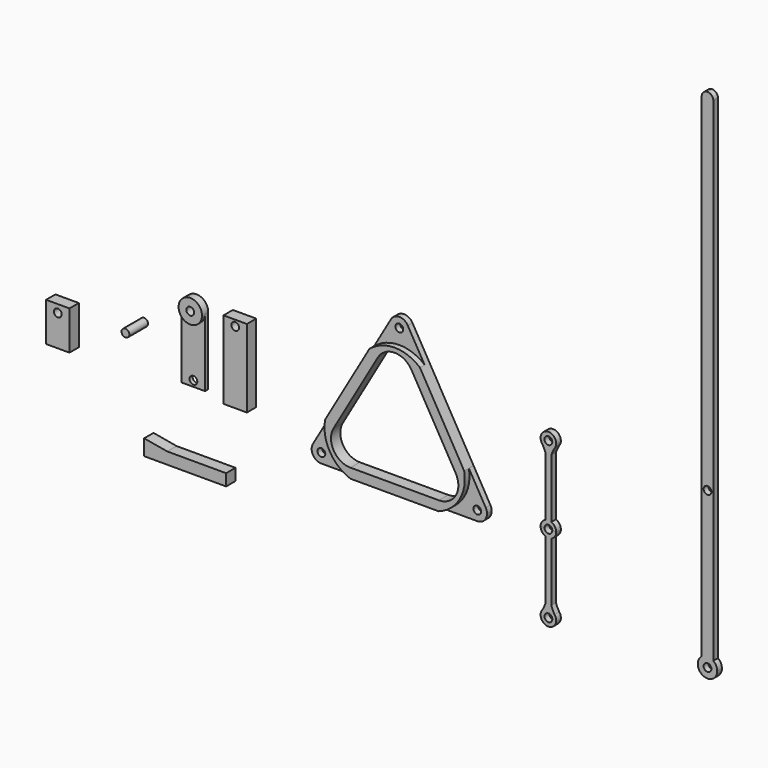
from build123d import *
from build123d import SkipClean  # not in build123d's __all__

# Parameters (mm, degrees)
F1_DEPTH  = 3
F0_R      = 1
F2_DEPTH  = 1.5
F4_DEPTH  = 1.5
F3_R      = 1
F5_DEPTH  = 1.5
F7_W      = 6
F7_H      = 20
F7_R      = 1
F8_DEPTH  = 3
F9_DEPTH  = 6
F10_DEPTH = 2
F11_DEPTH = 1
F12_R     = 1
F13_DEPTH = 1.5
F7_H_2    = 10
F14_DEPTH = 3
F16_DEPTH = 3


with BuildPart() as f1:
    # F0 (on Front) → F1 (new body)
    with BuildSketch(Plane.XZ):
        with BuildLine():
            Line((-33.1328085528, 8.75), (-44.4725545149, 28.3910161514))
            ThreePointArc((-44.4725545149, 28.3910161514), (-50.9677450433, 30.7875629885), (-57.4629355717, 28.3910161514))
            Line((-57.4629355717, 28.3910161514), (-68.8026815338, 8.75))
            ThreePointArc((-68.8026815338, 8.75), (-67.630556712, 1.9267265814), (-62.3074910055, -2.5))
            Line((-62.3074910055, -2.5), (-39.7018864751, -2.5))
            ThreePointArc((-39.7018864751, -2.5), (-34.3340694771, 1.9085363771), (-33.1328085528, 8.75))
        make_face()
        with BuildLine():
            Line((-39.6279990812, 0), (-62.3074910055, 0))
            ThreePointArc((-62.3074910055, 0), (-66.6376180244, 2.5), (-66.6376180244, 7.5))
            Line((-66.6376180244, 7.5), (-55.2978720622, 27.1410161514))
            ThreePointArc((-55.2978720622, 27.1410161514), (-50.9677450433, 29.6410161514), (-46.6376180244, 27.1410161514))
            Line((-46.6376180244, 27.1410161514), (-35.2978720622, 7.5))
            ThreePointArc((-35.2978720622, 7.5), (-35.2978720622, 2.5), (-39.6279990812, 0))
        make_face(mode=Mode.SUBTRACT)
    extrude(amount=F1_DEPTH)

    # F0 (on Front) → F2 (join)
    with BuildSketch(Plane.XZ):
        with BuildLine():
            ThreePointArc((-53.1328085528, 35.8910161514), (-51.6147926561, 32.2262015857), (-48.4677450433, 34.6410161514))
            ThreePointArc((-48.4677450433, 34.6410161514), (-48.5529304776, 35.2880637641), (-48.8026815338, 35.8910161514))
            ThreePointArc((-48.8026815338, 35.8910161514), (-50.9677450433, 37.1410161514), (-53.1328085528, 35.8910161514))
        make_face()
        with Locations((-50.9677450433, 34.6410161514)):
            Circle(F0_R, mode=Mode.SUBTRACT)
        with BuildLine():
            ThreePointArc((-48.8026815338, 35.8910161514), (-48.5529304776, 35.2880637641), (-48.4677450433, 34.6410161514))
            ThreePointArc((-48.4677450433, 34.6410161514), (-51.6147926561, 32.2262015857), (-53.1328085528, 35.8910161514))
            Line((-53.1328085528, 35.8910161514), (-57.4629355717, 28.3910161514))
            ThreePointArc((-57.4629355717, 28.3910161514), (-50.9677450433, 30.7875629885), (-44.4725545149, 28.3910161514))
            Line((-44.4725545149, 28.3910161514), (-48.8026815338, 35.8910161514))
        make_face()
        with BuildLine():
            Line((-28.8026815338, 1.25), (-33.1328085528, 8.75))
            ThreePointArc((-33.1328085528, 8.75), (-34.3340694771, 1.9085363771), (-39.7018864751, -2.5))
            Line((-39.7018864751, -2.5), (-30.9677450433, -2.5))
            ThreePointArc((-30.9677450433, -2.5), (-33.1328085528, 1.25), (-28.8026815338, 1.25))
        make_face()
        with BuildLine():
            ThreePointArc((-28.4677450433, 0), (-28.5529304776, 0.6470476128), (-28.8026815338, 1.25))
            ThreePointArc((-28.8026815338, 1.25), (-33.1328085528, 1.25), (-30.9677450433, -2.5))
            ThreePointArc((-30.9677450433, -2.5), (-29.1999780903, -1.767766953), (-28.4677450433, 0))
        make_face()
        with Locations((-30.9677450433, 0)):
            Circle(F0_R, mode=Mode.SUBTRACT)
        with BuildLine():
            ThreePointArc((-62.3074910055, -2.5), (-67.630556712, 1.9267265814), (-68.8026815338, 8.75))
            Line((-68.8026815338, 8.75), (-73.1328085528, 1.25))
            ThreePointArc((-73.1328085528, 1.25), (-70.3206974306, 2.4148145657), (-68.4677450433, 0))
            ThreePointArc((-68.4677450433, 0), (-69.1999780903, -1.767766953), (-70.9677450433, -2.5))
            Line((-70.9677450433, -2.5), (-62.3074910055, -2.5))
        make_face()
        with BuildLine():
            ThreePointArc((-68.4677450433, 0), (-70.3206974306, 2.4148145657), (-73.1328085528, 1.25))
            ThreePointArc((-73.1328085528, 1.25), (-73.1328085528, -1.25), (-70.9677450433, -2.5))
            ThreePointArc((-70.9677450433, -2.5), (-69.1999780903, -1.767766953), (-68.4677450433, 0))
        make_face()
        with Locations((-70.9677450433, 0)):
            Circle(F0_R, mode=Mode.SUBTRACT)
    extrude(amount=F2_DEPTH)


with BuildPart() as f4:
    # F3 (on Front) → F4 (new body)
    with BuildSketch(Plane.XZ):
        with BuildLine():
            Line((-11.9925050726, 18.5729119312), (-13.4582213502, 18.5729119312))
            Line((-13.4582213502, 18.5729119312), (-13.4582213502, 3.4791482928))
            ThreePointArc((-13.4582213502, 3.4791482928), (-14.3784990615, 2.7439302749), (-14.7253632114, 1.6182563162))
            Line((-14.7253632114, 1.6182563162), (-13.7253632114, 1.6182563162))
            ThreePointArc((-13.7253632114, 1.6182563162), (-12.7253632114, 2.6182563162), (-11.7253632114, 1.6182563162))
            Line((-11.7253632114, 1.6182563162), (-10.7253632114, 1.6182563162))
            ThreePointArc((-10.7253632114, 1.6182563162), (-11.0722273613, 2.7439302749), (-11.9925050726, 3.4791482928))
            Line((-11.9925050726, 3.4791482928), (-11.9925050726, 18.5729119312))
        make_face()
    extrude(amount=F4_DEPTH)

    # F3 (on Front) → F5 (join)
    with BuildSketch(Plane.XZ):
        with BuildLine():
            ThreePointArc((-14.3201244522, 20.4113028852), (-13.8423935019, 19.5140392553), (-13.4582213502, 18.5729119312))
            Line((-13.4582213502, 18.5729119312), (-11.9925050726, 18.5729119312))
            ThreePointArc((-11.9925050726, 18.5729119312), (-11.6083329209, 19.5140392553), (-11.1306019706, 20.4113028852))
            ThreePointArc((-11.1306019706, 20.4113028852), (-12.7253632114, 23.6182563162), (-14.3201244522, 20.4113028852))
        make_face()
        with Locations((-12.7253632114, 21.6182563162)):
            Circle(F3_R, mode=Mode.SUBTRACT)
    extrude(amount=F5_DEPTH)

    # F6: F4 across face


with BuildPart() as f4_1:
    add(f4.part, clean=False)
    with SkipClean():  # cleaning this boolean's faces spoils the solid; the shape is the same uncleaned
        add(f4.part.mirror(Plane(origin=(-14.2253632114, -0.75, 1.6182563162), x_dir=(1, 0, 0), z_dir=(0, 0, -1))), clean=False)


with BuildPart() as f8:
    # F7 (on Front) → F8 (new body)
    with BuildSketch(Plane.XZ):
        with Locations((-91.8792099953, 13.8065970875)):
            Rectangle(F7_W, F7_H)
        with Locations((-91.8792099953, 22.3065970875)):
            Circle(F7_R, mode=Mode.SUBTRACT)
    extrude(amount=F8_DEPTH)


with BuildPart() as f9:
    # F7 (on Front) → F9 (new body)
    with BuildSketch(Plane.XZ):
        with Locations((-117.6395714283, 13.6291719973)):
            Circle(F7_R)
    extrude(amount=F9_DEPTH)


with BuildPart() as f10:
    # F7 (on Front) → F10 (new body)
    with BuildSketch(Plane.XZ):
        with BuildLine():
            ThreePointArc((-107.204214007, 21.3065970875), (-104.204214007, 18.3065970875), (-101.204214007, 21.3065970875))
            Line((-101.204214007, 21.3065970875), (-103.204214007, 21.3065970875))
            ThreePointArc((-103.204214007, 21.3065970875), (-104.204214007, 20.3065970875), (-105.204214007, 21.3065970875))
            Line((-105.204214007, 21.3065970875), (-107.204214007, 21.3065970875))
        make_face()
        with BuildLine():
            Line((-103.204214007, 21.3065970875), (-101.204214007, 21.3065970875))
            ThreePointArc((-101.204214007, 21.3065970875), (-104.204214007, 24.3065970875), (-107.204214007, 21.3065970875))
            Line((-107.204214007, 21.3065970875), (-105.204214007, 21.3065970875))
            ThreePointArc((-105.204214007, 21.3065970875), (-104.204214007, 22.3065970875), (-103.204214007, 21.3065970875))
        make_face()
    extrude(amount=F10_DEPTH)

    # F7 (on Front) → F11 (join)
    with BuildSketch(Plane.XZ):
        with BuildLine():
            Line((-101.204214007, 3.8065970875), (-101.204214007, 21.3065970875))
            ThreePointArc((-101.204214007, 21.3065970875), (-104.204214007, 18.3065970875), (-107.204214007, 21.3065970875))
            Line((-107.204214007, 21.3065970875), (-107.204214007, 3.8065970875))
            Line((-107.204214007, 3.8065970875), (-101.204214007, 3.8065970875))
        make_face()
        with Locations((-104.204214007, 5.3065970875)):
            Circle(F7_R, mode=Mode.SUBTRACT)
    extrude(amount=F11_DEPTH)


with BuildPart() as f13:
    # F12 (on Front) → F13 (new body)
    with BuildSketch(Plane.XZ):
        with BuildLine():
            ThreePointArc((26.5937472323, -14.345602423), (28.0937472323, -13.845602423), (29.5937472323, -14.345602423))
            Line((29.5937472323, -14.345602423), (29.5937472323, 112.154397577))
            ThreePointArc((29.5937472323, 112.154397577), (29.1544074041, 113.2150577488), (28.0937472323, 113.654397577))
            ThreePointArc((28.0937472323, 113.654397577), (27.0330870605, 113.2150577488), (26.5937472323, 112.154397577))
            Line((26.5937472323, 112.154397577), (26.5937472323, -14.345602423))
        make_face()
        with Locations((28.0937472323, 23.654397577)):
            Circle(F12_R, mode=Mode.SUBTRACT)
        with BuildLine():
            Line((29.5937472323, -14.345602423), (29.5937472323, -16.345602423))
            Line((29.5937472323, -16.345602423), (29.0937472323, -16.345602423))
            ThreePointArc((29.0937472323, -16.345602423), (28.0937472323, -17.345602423), (27.0937472323, -16.345602423))
            Line((27.0937472323, -16.345602423), (26.5937472323, -16.345602423))
            Line((26.5937472323, -16.345602423), (26.5937472323, -14.345602423))
            ThreePointArc((26.5937472323, -14.345602423), (26.9757132436, -18.5816704005), (30.5937472323, -16.345602423))
            ThreePointArc((30.5937472323, -16.345602423), (30.3298152098, -15.2275684342), (29.5937472323, -14.345602423))
        make_face()
        with BuildLine():
            Line((29.0937472323, -16.345602423), (29.5937472323, -16.345602423))
            Line((29.5937472323, -16.345602423), (29.5937472323, -14.345602423))
            ThreePointArc((29.5937472323, -14.345602423), (28.0937472323, -13.845602423), (26.5937472323, -14.345602423))
            Line((26.5937472323, -14.345602423), (26.5937472323, -16.345602423))
            Line((26.5937472323, -16.345602423), (27.0937472323, -16.345602423))
            ThreePointArc((27.0937472323, -16.345602423), (28.0937472323, -15.345602423), (29.0937472323, -16.345602423))
        make_face()
    extrude(amount=F13_DEPTH)


with BuildPart() as f14:
    # F7 (on Front) → F14 (new body)
    with BuildSketch(Plane.XZ):
        with Locations((-137.3983682394, 7.5233563501)):
            Rectangle(F7_W, F7_H_2)
        with Locations((-137.3983682394, 10.5233563501)):
            Circle(F7_R, mode=Mode.SUBTRACT)
    extrude(amount=F14_DEPTH)


with BuildPart() as f16:
    # F15 (on Front) → F16 (new body)
    with BuildSketch(Plane.XZ):
        Polygon((-94.2028054563, -11.6239395214), (-109.3253716573, -11.6239395214), (-115.2342181754, -10.5820504554), (-115.2342181754, -14.6239395214), (-109.2342181754, -14.6239395214), (-94.2028054563, -14.6239395214), align=None)
    extrude(amount=F16_DEPTH)


solid = Compound([f1.part, f4_1.part, f8.part, f9.part, f10.part, f13.part, f14.part, f16.part])
